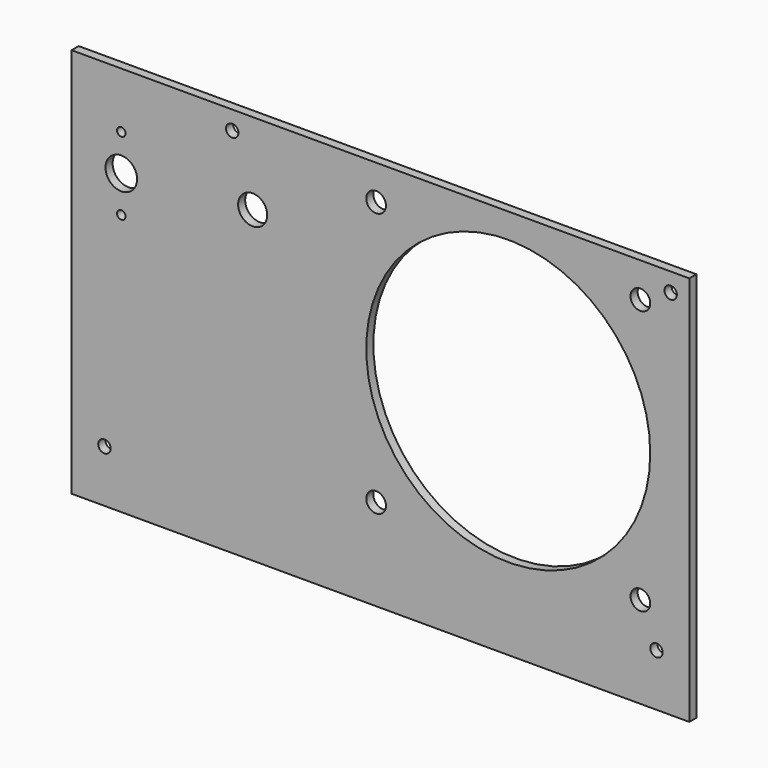
from build123d import *

# Parameters (mm, degrees)
F0_W     = 174
F0_H     = 110
F0_R     = 1.75
F0_R_2   = 2.778
F0_R_3   = 1.2
F0_R_4   = 4.45
F0_R_5   = 4.1
F0_R_6   = 40
F1_DEPTH = 2.5


# Not quite as in the source:
# - a feature names something its author has since deleted; it is built from what else it names


with BuildPart() as f1:
    # F0 (on Front) → F1 (new body)
    with BuildSketch(Plane.XZ):
        Rectangle(F0_W, F0_H)
        with Locations((-77.75, -40.25)):
            Circle(F0_R, mode=Mode.SUBTRACT)
        with Locations((-1.222, -29.222)):
            Circle(F0_R_2, mode=Mode.SUBTRACT)
        with Locations((77.75, -40.25)):
            Circle(F0_R, mode=Mode.SUBTRACT)
        with Locations((73.222, -29.222)):
            Circle(F0_R_2, mode=Mode.SUBTRACT)
        with Locations((-73, 18.7)):
            Circle(F0_R_3, mode=Mode.SUBTRACT)
        with Locations((-73, 29)):
            Circle(F0_R_4, mode=Mode.SUBTRACT)
        with Locations((-73, 39.3)):
            Circle(F0_R_3, mode=Mode.SUBTRACT)
        with Locations((-36, 32)):
            Circle(F0_R_5, mode=Mode.SUBTRACT)
        with Locations((-41.75, 49.75)):
            Circle(F0_R, mode=Mode.SUBTRACT)
        with Locations((-1.222, 45.222)):
            Circle(F0_R_2, mode=Mode.SUBTRACT)
        with Locations((36, 8)):
            Circle(F0_R_6, mode=Mode.SUBTRACT)
        with Locations((73.222, 45.222)):
            Circle(F0_R_2, mode=Mode.SUBTRACT)
        with Locations((81.75, 49.75)):
            Circle(F0_R, mode=Mode.SUBTRACT)
    extrude(amount=F1_DEPTH)


solid = f1.part
